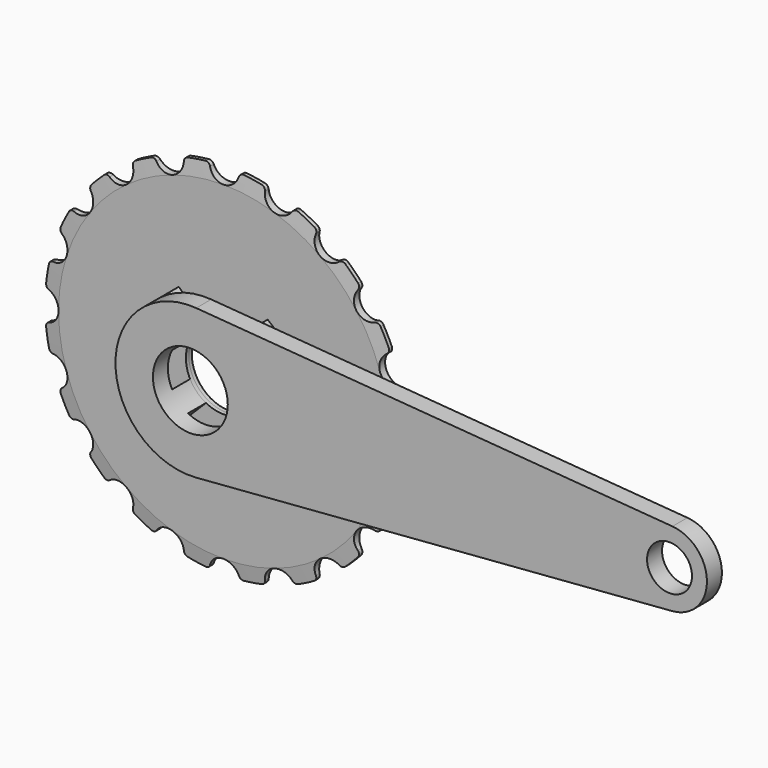
from build123d import *
from build123d import SkipClean  # not in build123d's __all__

# Parameters (mm, degrees)
F2_R          = 6.35
F3_DEPTH      = 1.5885
F3_DEPTH_BACK = 1.5885
F4_T1_DEPTH   = 10.5199898753
F5_R          = 15.875
F6_DEPTH      = 1.5885001
F6_DEPTH_BACK = 1.5885001
F8_D          = 5
F10_R         = 15.875
F10_R_2       = 9.525
F11_DEPTH     = 17.4625
F12_R         = 9.525
F12_R_2       = 15.875
F13_DEPTH     = 9.525
F15_DEPTH     = 9.525


# Not quite as in the source:
# - a fillet or chamfer that OpenCascade refuses, or shapes differently, is made with other operations: its cross-section is extruded or revolved along the edge and cut away or added


with BuildPart() as f1:
    # F0 (on Right) → F1 (revolve)
    with BuildSketch(Plane.YZ):
        Polygon((-0.79375, 76.2), (-1.5875, 69.85), (-1.5875, 0), (1.5875, 0), (1.5875, 69.85), (0.79375, 76.2), (0, 76.2), align=None)
    revolve(axis=Axis((0, -19.5679962635, 0), (0, -1, 0)))

    # F2 (on Front) → F3 (cut, two sides)
    with BuildSketch(Plane.XZ) as f3_sk:
        with Locations((0, 76.2)):
            Circle(F2_R)
        with Locations((-23.5470949714, 72.4705065417)):
            Circle(F2_R)
        with Locations((-44.7892362247, 61.6470949714)):
            Circle(F2_R)
        with Locations((-61.6470949714, 44.7892362247)):
            Circle(F2_R)
        with Locations((-72.4705065417, 23.5470949714)):
            Circle(F2_R)
        with Locations((-76.2, 0)):
            Circle(F2_R)
        with Locations((-72.4705065417, -23.5470949714)):
            Circle(F2_R)
        with Locations((-61.6470949714, -44.7892362247)):
            Circle(F2_R)
        with Locations((-44.7892362247, -61.6470949714)):
            Circle(F2_R)
        with Locations((-23.5470949714, -72.4705065417)):
            Circle(F2_R)
        with Locations((0, -76.2)):
            Circle(F2_R)
        with Locations((23.5470949714, -72.4705065417)):
            Circle(F2_R)
        with Locations((44.7892362247, -61.6470949714)):
            Circle(F2_R)
        with Locations((61.6470949714, -44.7892362247)):
            Circle(F2_R)
        with Locations((72.4705065417, -23.5470949714)):
            Circle(F2_R)
        with Locations((76.2, 0)):
            Circle(F2_R)
        with Locations((72.4705065417, 23.5470949714)):
            Circle(F2_R)
        with Locations((61.6470949714, 44.7892362247)):
            Circle(F2_R)
        with Locations((44.7892362247, 61.6470949714)):
            Circle(F2_R)
        with Locations((23.5470949714, 72.4705065417)):
            Circle(F2_R)
    extrude(amount=-F3_DEPTH, mode=Mode.SUBTRACT)
    extrude(f3_sk.sketch, amount=F3_DEPTH_BACK, mode=Mode.SUBTRACT)

    # F4: fillet of radius 1.905 on 40 edges, made by hand

    # F4_s2 → F4_t1 (cut)
    with BuildSketch(Plane.XZ.offset(-5.2599949376)):
        with BuildLine():
            ThreePointArc((-31.1382740919, 69.5474506116), (-29.8427555478, 69.6422506994), (-28.7876505623, 68.8845510068))
            ThreePointArc((-28.7876505623, 68.8845510068), (-29.185470054, 69.5496802154), (-29.4992984573, 70.258319013))
            ThreePointArc((-29.4992984573, 70.258319013), (-30.320869622, 69.9076881706), (-31.1382740919, 69.5474506116))
        make_face()
        with BuildLine():
            ThreePointArc((-17.1996246595, 72.6497288631), (-16.7913915004, 73.8828959411), (-15.6875728882, 74.5676877533))
            ThreePointArc((-15.6875728882, 74.5676877533), (-16.5606093201, 74.378667768), (-17.4313699926, 74.1794266639))
            ThreePointArc((-17.4313699926, 74.1794266639), (-17.2687350698, 73.4216621266), (-17.1996246595, 72.6497288631))
        make_face()
        with BuildLine():
            ThreePointArc((8.1229143268, 75.7658119658), (6.8615081353, 75.4556349604), (6.0921857451, 74.408974359))
            ThreePointArc((6.0921857451, 74.408974359), (6.264998336, 75.1644828106), (6.3444854527, 75.9354166667))
            ThreePointArc((6.3444854527, 75.9354166667), (7.2341969516, 75.8558263713), (8.1229143268, 75.7658119658))
        make_face()
        with BuildLine():
            ThreePointArc((-8.1229143268, 75.7658119658), (-6.8615081353, 75.4556349604), (-6.0921857451, 74.408974359))
            ThreePointArc((-6.0921857451, 74.408974359), (-6.264998336, 75.1644828106), (-6.3444854527, 75.9354166667))
            ThreePointArc((-6.3444854527, 75.9354166667), (-7.2341969516, 75.8558263713), (-8.1229143268, 75.7658119658))
        make_face()
        with BuildLine():
            ThreePointArc((-51.1056026357, 56.521300226), (-49.9027861206, 57.0117977139), (-48.6651795671, 56.6172278552))
            ThreePointArc((-48.6651795671, 56.6172278552), (-49.2490646159, 57.1268703396), (-49.7665145952, 57.7038475758))
            ThreePointArc((-49.7665145952, 57.7038475758), (-50.439524316, 57.1164983764), (-51.1056026357, 56.521300226))
        make_face()
        with BuildLine():
            ThreePointArc((-38.8078159657, 63.7790217256), (-38.8006327436, 65.0779842948), (-37.9624511672, 66.0703587199))
            ThreePointArc((-37.9624511672, 66.0703587199), (-38.734347767, 65.620806937), (-39.5009214915, 65.1622375408))
            ThreePointArc((-39.5009214915, 65.1622375408), (-39.1120843687, 64.4918175948), (-38.8078159657, 63.7790217256))
        make_face()
        with BuildLine():
            ThreePointArc((28.7876505623, 68.8845510068), (29.8427555478, 69.6422506994), (31.1382740919, 69.5474506116))
            ThreePointArc((31.1382740919, 69.5474506116), (30.320869622, 69.9076881706), (29.4992984573, 70.258319013))
            ThreePointArc((29.4992984573, 70.258319013), (29.185470054, 69.5496802154), (28.7876505623, 68.8845510068))
        make_face()
        with BuildLine():
            ThreePointArc((17.1996246595, 72.6497288631), (16.7913915004, 73.8828959411), (15.6875728882, 74.5676877533))
            ThreePointArc((15.6875728882, 74.5676877533), (16.5606093201, 74.378667768), (17.4313699926, 74.1794266639))
            ThreePointArc((17.4313699926, 74.1794266639), (17.2687350698, 73.4216621266), (17.1996246595, 72.6497288631))
        make_face()
        with BuildLine():
            ThreePointArc((48.6651795671, 56.6172278552), (49.9027861206, 57.0117977139), (51.1056026357, 56.521300226))
            ThreePointArc((51.1056026357, 56.521300226), (50.439524316, 57.1164983764), (49.7665145952, 57.7038475758))
            ThreePointArc((49.7665145952, 57.7038475758), (49.2490646159, 57.1268703396), (48.6651795671, 56.6172278552))
        make_face()
        with BuildLine():
            ThreePointArc((38.8078159657, 63.7790217256), (38.8006327436, 65.0779842948), (37.9624511672, 66.0703587199))
            ThreePointArc((37.9624511672, 66.0703587199), (38.734347767, 65.620806937), (39.5009214915, 65.1622375408))
            ThreePointArc((39.5009214915, 65.1622375408), (39.1120843687, 64.4918175948), (38.8078159657, 63.7790217256))
        make_face()
        with BuildLine():
            ThreePointArc((56.521300226, 51.1056026357), (57.0117977139, 49.9027861206), (56.6172278552, 48.6651795671))
            ThreePointArc((56.6172278552, 48.6651795671), (57.1268703396, 49.2490646159), (57.7038475758, 49.7665145952))
            ThreePointArc((57.7038475758, 49.7665145952), (57.1164983764, 50.439524316), (56.521300226, 51.1056026357))
        make_face()
        with BuildLine():
            ThreePointArc((63.7790217256, 38.8078159657), (65.0779842948, 38.8006327436), (66.0703587199, 37.9624511672))
            ThreePointArc((66.0703587199, 37.9624511672), (65.620806937, 38.734347767), (65.1622375408, 39.5009214915))
            ThreePointArc((65.1622375408, 39.5009214915), (64.4918175948, 39.1120843687), (63.7790217256, 38.8078159657))
        make_face()
        with BuildLine():
            ThreePointArc((-66.0703587199, 37.9624511672), (-65.0779842948, 38.8006327436), (-63.7790217256, 38.8078159657))
            ThreePointArc((-63.7790217256, 38.8078159657), (-64.4918175948, 39.1120843687), (-65.1622375408, 39.5009214915))
            ThreePointArc((-65.1622375408, 39.5009214915), (-65.620806937, 38.734347767), (-66.0703587199, 37.9624511672))
        make_face()
        with BuildLine():
            ThreePointArc((-56.6172278552, 48.6651795671), (-57.0117977139, 49.9027861206), (-56.521300226, 51.1056026357))
            ThreePointArc((-56.521300226, 51.1056026357), (-57.1164983764, 50.439524316), (-57.7038475758, 49.7665145952))
            ThreePointArc((-57.7038475758, 49.7665145952), (-57.1268703396, 49.2490646159), (-56.6172278552, 48.6651795671))
        make_face()
        with BuildLine():
            ThreePointArc((-74.5676877533, 15.6875728882), (-73.8828959411, 16.7913915004), (-72.6497288631, 17.1996246595))
            ThreePointArc((-72.6497288631, 17.1996246595), (-73.4216621266, 17.2687350698), (-74.1794266639, 17.4313699926))
            ThreePointArc((-74.1794266639, 17.4313699926), (-74.378667768, 16.5606093201), (-74.5676877533, 15.6875728882))
        make_face()
        with BuildLine():
            ThreePointArc((-68.8845510068, 28.7876505623), (-69.6422506994, 29.8427555478), (-69.5474506116, 31.1382740919))
            ThreePointArc((-69.5474506116, 31.1382740919), (-69.9076881706, 30.320869622), (-70.258319013, 29.4992984573))
            ThreePointArc((-70.258319013, 29.4992984573), (-69.5496802154, 29.185470054), (-68.8845510068, 28.7876505623))
        make_face()
        with BuildLine():
            ThreePointArc((-75.7658119658, -8.1229143268), (-75.4556349604, -6.8615081353), (-74.408974359, -6.0921857451))
            ThreePointArc((-74.408974359, -6.0921857451), (-75.1644828106, -6.264998336), (-75.9354166667, -6.3444854527))
            ThreePointArc((-75.9354166667, -6.3444854527), (-75.8558263713, -7.2341969516), (-75.7658119658, -8.1229143268))
        make_face()
        with BuildLine():
            ThreePointArc((-74.408974359, 6.0921857451), (-75.4556349604, 6.8615081353), (-75.7658119658, 8.1229143268))
            ThreePointArc((-75.7658119658, 8.1229143268), (-75.8558263713, 7.2341969516), (-75.9354166667, 6.3444854527))
            ThreePointArc((-75.9354166667, 6.3444854527), (-75.1644828106, 6.264998336), (-74.408974359, 6.0921857451))
        make_face()
        with BuildLine():
            ThreePointArc((-69.5474506116, -31.1382740919), (-69.6422506994, -29.8427555478), (-68.8845510068, -28.7876505623))
            ThreePointArc((-68.8845510068, -28.7876505623), (-69.5496802154, -29.185470054), (-70.258319013, -29.4992984573))
            ThreePointArc((-70.258319013, -29.4992984573), (-69.9076881706, -30.320869622), (-69.5474506116, -31.1382740919))
        make_face()
        with BuildLine():
            ThreePointArc((-72.6497288631, -17.1996246595), (-73.8828959411, -16.7913915004), (-74.5676877533, -15.6875728882))
            ThreePointArc((-74.5676877533, -15.6875728882), (-74.378667768, -16.5606093201), (-74.1794266639, -17.4313699926))
            ThreePointArc((-74.1794266639, -17.4313699926), (-73.4216621266, -17.2687350698), (-72.6497288631, -17.1996246595))
        make_face()
        with BuildLine():
            ThreePointArc((-56.521300226, -51.1056026357), (-57.0117977139, -49.9027861206), (-56.6172278552, -48.6651795671))
            ThreePointArc((-56.6172278552, -48.6651795671), (-57.1268703396, -49.2490646159), (-57.7038475758, -49.7665145952))
            ThreePointArc((-57.7038475758, -49.7665145952), (-57.1164983764, -50.439524316), (-56.521300226, -51.1056026357))
        make_face()
        with BuildLine():
            ThreePointArc((-63.7790217256, -38.8078159657), (-65.0779842948, -38.8006327436), (-66.0703587199, -37.9624511672))
            ThreePointArc((-66.0703587199, -37.9624511672), (-65.620806937, -38.734347767), (-65.1622375408, -39.5009214915))
            ThreePointArc((-65.1622375408, -39.5009214915), (-64.4918175948, -39.1120843687), (-63.7790217256, -38.8078159657))
        make_face()
        with BuildLine():
            ThreePointArc((-37.9624511672, -66.0703587199), (-38.8006327436, -65.0779842948), (-38.8078159657, -63.7790217256))
            ThreePointArc((-38.8078159657, -63.7790217256), (-39.1120843687, -64.4918175948), (-39.5009214915, -65.1622375408))
            ThreePointArc((-39.5009214915, -65.1622375408), (-38.734347767, -65.620806937), (-37.9624511672, -66.0703587199))
        make_face()
        with BuildLine():
            ThreePointArc((-48.6651795671, -56.6172278552), (-49.9027861206, -57.0117977139), (-51.1056026357, -56.521300226))
            ThreePointArc((-51.1056026357, -56.521300226), (-50.439524316, -57.1164983764), (-49.7665145952, -57.7038475758))
            ThreePointArc((-49.7665145952, -57.7038475758), (-49.2490646159, -57.1268703396), (-48.6651795671, -56.6172278552))
        make_face()
        with BuildLine():
            ThreePointArc((-15.6875728882, -74.5676877533), (-16.7913915004, -73.8828959411), (-17.1996246595, -72.6497288631))
            ThreePointArc((-17.1996246595, -72.6497288631), (-17.2687350698, -73.4216621266), (-17.4313699926, -74.1794266639))
            ThreePointArc((-17.4313699926, -74.1794266639), (-16.5606093201, -74.378667768), (-15.6875728882, -74.5676877533))
        make_face()
        with BuildLine():
            ThreePointArc((-28.7876505623, -68.8845510068), (-29.8427555478, -69.6422506994), (-31.1382740919, -69.5474506116))
            ThreePointArc((-31.1382740919, -69.5474506116), (-30.320869622, -69.9076881706), (-29.4992984573, -70.258319013))
            ThreePointArc((-29.4992984573, -70.258319013), (-29.185470054, -69.5496802154), (-28.7876505623, -68.8845510068))
        make_face()
        with BuildLine():
            ThreePointArc((8.1229143268, -75.7658119658), (6.8615081353, -75.4556349604), (6.0921857451, -74.408974359))
            ThreePointArc((6.0921857451, -74.408974359), (6.264998336, -75.1644828106), (6.3444854527, -75.9354166667))
            ThreePointArc((6.3444854527, -75.9354166667), (7.2341969516, -75.8558263713), (8.1229143268, -75.7658119658))
        make_face()
        with BuildLine():
            ThreePointArc((-6.0921857451, -74.408974359), (-6.8615081353, -75.4556349604), (-8.1229143268, -75.7658119658))
            ThreePointArc((-8.1229143268, -75.7658119658), (-7.2341969516, -75.8558263713), (-6.3444854527, -75.9354166667))
            ThreePointArc((-6.3444854527, -75.9354166667), (-6.264998336, -75.1644828106), (-6.0921857451, -74.408974359))
        make_face()
        with BuildLine():
            ThreePointArc((31.1382740919, -69.5474506116), (29.8427555478, -69.6422506994), (28.7876505623, -68.8845510068))
            ThreePointArc((28.7876505623, -68.8845510068), (29.185470054, -69.5496802154), (29.4992984573, -70.258319013))
            ThreePointArc((29.4992984573, -70.258319013), (30.320869622, -69.9076881706), (31.1382740919, -69.5474506116))
        make_face()
        with BuildLine():
            ThreePointArc((17.1996246595, -72.6497288631), (16.7913915004, -73.8828959411), (15.6875728882, -74.5676877533))
            ThreePointArc((15.6875728882, -74.5676877533), (16.5606093201, -74.378667768), (17.4313699926, -74.1794266639))
            ThreePointArc((17.4313699926, -74.1794266639), (17.2687350698, -73.4216621266), (17.1996246595, -72.6497288631))
        make_face()
        with BuildLine():
            ThreePointArc((51.1056026357, -56.521300226), (49.9027861206, -57.0117977139), (48.6651795671, -56.6172278552))
            ThreePointArc((48.6651795671, -56.6172278552), (49.2490646159, -57.1268703396), (49.7665145952, -57.7038475758))
            ThreePointArc((49.7665145952, -57.7038475758), (50.439524316, -57.1164983764), (51.1056026357, -56.521300226))
        make_face()
        with BuildLine():
            ThreePointArc((38.8078159657, -63.7790217256), (38.8006327436, -65.0779842948), (37.9624511672, -66.0703587199))
            ThreePointArc((37.9624511672, -66.0703587199), (38.734347767, -65.620806937), (39.5009214915, -65.1622375408))
            ThreePointArc((39.5009214915, -65.1622375408), (39.1120843687, -64.4918175948), (38.8078159657, -63.7790217256))
        make_face()
        with BuildLine():
            ThreePointArc((66.0703587199, -37.9624511672), (65.0779842948, -38.8006327436), (63.7790217256, -38.8078159657))
            ThreePointArc((63.7790217256, -38.8078159657), (64.4918175948, -39.1120843687), (65.1622375408, -39.5009214915))
            ThreePointArc((65.1622375408, -39.5009214915), (65.620806937, -38.734347767), (66.0703587199, -37.9624511672))
        make_face()
        with BuildLine():
            ThreePointArc((56.6172278552, -48.6651795671), (57.0117977139, -49.9027861206), (56.521300226, -51.1056026357))
            ThreePointArc((56.521300226, -51.1056026357), (57.1164983764, -50.439524316), (57.7038475758, -49.7665145952))
            ThreePointArc((57.7038475758, -49.7665145952), (57.1268703396, -49.2490646159), (56.6172278552, -48.6651795671))
        make_face()
        with BuildLine():
            ThreePointArc((74.5676877533, -15.6875728882), (73.8828959411, -16.7913915004), (72.6497288631, -17.1996246595))
            ThreePointArc((72.6497288631, -17.1996246595), (73.4216621266, -17.2687350698), (74.1794266639, -17.4313699926))
            ThreePointArc((74.1794266639, -17.4313699926), (74.378667768, -16.5606093201), (74.5676877533, -15.6875728882))
        make_face()
        with BuildLine():
            ThreePointArc((68.8845510068, -28.7876505623), (69.6422506994, -29.8427555478), (69.5474506116, -31.1382740919))
            ThreePointArc((69.5474506116, -31.1382740919), (69.9076881706, -30.320869622), (70.258319013, -29.4992984573))
            ThreePointArc((70.258319013, -29.4992984573), (69.5496802154, -29.185470054), (68.8845510068, -28.7876505623))
        make_face()
        with BuildLine():
            ThreePointArc((69.5474506116, 31.1382740919), (69.6422506994, 29.8427555478), (68.8845510068, 28.7876505623))
            ThreePointArc((68.8845510068, 28.7876505623), (69.5496802154, 29.185470054), (70.258319013, 29.4992984573))
            ThreePointArc((70.258319013, 29.4992984573), (69.9076881706, 30.320869622), (69.5474506116, 31.1382740919))
        make_face()
        with BuildLine():
            ThreePointArc((72.6497288631, 17.1996246595), (73.8828959411, 16.7913915004), (74.5676877533, 15.6875728882))
            ThreePointArc((74.5676877533, 15.6875728882), (74.378667768, 16.5606093201), (74.1794266639, 17.4313699926))
            ThreePointArc((74.1794266639, 17.4313699926), (73.4216621266, 17.2687350698), (72.6497288631, 17.1996246595))
        make_face()
        with BuildLine():
            ThreePointArc((75.7658119658, 8.1229143268), (75.4556349604, 6.8615081353), (74.408974359, 6.0921857451))
            ThreePointArc((74.408974359, 6.0921857451), (75.1644828106, 6.264998336), (75.9354166667, 6.3444854527))
            ThreePointArc((75.9354166667, 6.3444854527), (75.8558263713, 7.2341969516), (75.7658119658, 8.1229143268))
        make_face()
        with BuildLine():
            ThreePointArc((74.408974359, -6.0921857451), (75.4556349604, -6.8615081353), (75.7658119658, -8.1229143268))
            ThreePointArc((75.7658119658, -8.1229143268), (75.8558263713, -7.2341969516), (75.9354166667, -6.3444854527))
            ThreePointArc((75.9354166667, -6.3444854527), (75.1644828106, -6.264998336), (74.408974359, -6.0921857451))
        make_face()
    extrude(amount=F4_T1_DEPTH, mode=Mode.SUBTRACT)

    # F5 (on Front) → F6 (cut, two sides)
    with BuildSketch(Plane.XZ) as f6_sk:
        Circle(F5_R)
    extrude(amount=-F6_DEPTH, mode=Mode.SUBTRACT)
    extrude(f6_sk.sketch, amount=F6_DEPTH_BACK, mode=Mode.SUBTRACT)

    # F8 (through all)
    with Locations(Plane.XZ.offset(1.5875)):
        with Locations((-17.9605122421, 17.9605122421), (17.9605122421, 17.9605122421), (17.9605122421, -17.9605122421), (-17.9605122421, -17.9605122421)):
            Hole(F8_D / 2)


with BuildPart() as f11:
    # F10 (on offset) → F11 (new body, through all)
    with BuildSketch(Plane.XZ.offset(19.05)):
        with BuildLine():
            ThreePointArc((2.48046875, -31.6529583891), (23.3111280595, -21.5558300372), (31.75, 0))
            ThreePointArc((31.75, 0), (23.3111280595, 21.5558300372), (2.48046875, 31.6529583891))
            ThreePointArc((2.48046875, 31.6529583891), (-31.75, 0), (2.48046875, -31.6529583891))
        make_face()
        Circle(F10_R, mode=Mode.SUBTRACT)
        with BuildLine():
            ThreePointArc((2.48046875, 31.6529583891), (23.3111280595, 21.5558300372), (31.75, 0))
            ThreePointArc((31.75, 0), (23.3111280595, -21.5558300372), (2.48046875, -31.6529583891))
            Line((2.48046875, -31.6529583891), (204.440234375, -15.8264791945))
            ThreePointArc((204.440234375, -15.8264791945), (187.325, 0), (204.440234375, 15.8264791945))
            Line((204.440234375, 15.8264791945), (2.48046875, 31.6529583891))
        make_face()
        with BuildLine():
            ThreePointArc((219.075, 0), (214.8555640297, 10.7779150186), (204.440234375, 15.8264791945))
            ThreePointArc((204.440234375, 15.8264791945), (187.325, 0), (204.440234375, -15.8264791945))
            ThreePointArc((204.440234375, -15.8264791945), (214.8555640297, -10.7779150186), (219.075, 0))
        make_face()
        with Locations((203.2, 0)):
            Circle(F10_R_2, mode=Mode.SUBTRACT)
    extrude(amount=-F11_DEPTH)

    # F12 (on face) → F13 (cut)
    with BuildSketch(Plane(origin=(0, -1.5875, 0), x_dir=(-1, 0, 0), z_dir=(0, 1, 0))):
        with BuildLine():
            Line((-2.48046875, 31.6529583891), (-204.440234375, 15.8264791945))
            ThreePointArc((-204.440234375, 15.8264791945), (-187.325, 0), (-204.440234375, -15.8264791945))
            Line((-204.440234375, -15.8264791945), (-2.48046875, -31.6529583891))
            ThreePointArc((-2.48046875, -31.6529583891), (-31.75, 0), (-2.48046875, 31.6529583891))
        make_face()
        with BuildLine():
            ThreePointArc((-204.440234375, -15.8264791945), (-187.325, 0), (-204.440234375, 15.8264791945))
            ThreePointArc((-204.440234375, 15.8264791945), (-219.075, 0), (-204.440234375, -15.8264791945))
        make_face()
        with Locations((-203.2, 0)):
            Circle(F12_R, mode=Mode.SUBTRACT)
        Circle(F12_R_2)
        with Locations((-203.2, 0)):
            Circle(F12_R)
    with SkipClean():  # cleaning this boolean's faces spoils the solid; the shape is the same uncleaned
        extrude(amount=-F13_DEPTH, mode=Mode.SUBTRACT)

    # F14 (on face) → F15 (cut, through all)
    with BuildSketch(Plane(origin=(0, -1.5875, 0), x_dir=(-1, 0, 0), z_dir=(0, 1, 0))):
        with BuildLine():
            ThreePointArc((-7.3406768954, 14.0758689862), (0, 15.875), (7.3406768954, 14.0758689862))
            Line((7.3406768954, 14.0758689862), (18.829037638, 25.5642297288))
            ThreePointArc((18.829037638, 25.5642297288), (8.7227908576, 30.5282724643), (-2.48046875, 31.6529583891))
            ThreePointArc((-2.48046875, 31.6529583891), (-11.0811515557, 29.7534969407), (-18.829037638, 25.5642297288))
            Line((-18.829037638, 25.5642297288), (-7.3406768954, 14.0758689862))
        make_face()
        with BuildLine():
            ThreePointArc((-15.875, 0), (-15.4186582613, 3.7789684336), (-14.0758689862, 7.3406768954))
            Line((-14.0758689862, 7.3406768954), (-25.5642297288, 18.829037638))
            ThreePointArc((-25.5642297288, 18.829037638), (-31.75, 0), (-25.5642297288, -18.829037638))
            Line((-25.5642297288, -18.829037638), (-14.0758689862, -7.3406768954))
            ThreePointArc((-14.0758689862, -7.3406768954), (-15.4186582613, -3.7789684336), (-15.875, 0))
        make_face()
        with BuildLine():
            Line((18.829037638, -25.5642297288), (7.3406768954, -14.0758689862))
            ThreePointArc((7.3406768954, -14.0758689862), (0, -15.875), (-7.3406768954, -14.0758689862))
            Line((-7.3406768954, -14.0758689862), (-18.829037638, -25.5642297288))
            ThreePointArc((-18.829037638, -25.5642297288), (-11.0811515557, -29.7534969407), (-2.48046875, -31.6529583891))
            ThreePointArc((-2.48046875, -31.6529583891), (8.7227908576, -30.5282724643), (18.829037638, -25.5642297288))
        make_face()
        with BuildLine():
            ThreePointArc((14.0758689862, 7.3406768954), (15.4186582613, 3.7789684336), (15.875, 0))
            ThreePointArc((15.875, 0), (15.4186582613, -3.7789684336), (14.0758689862, -7.3406768954))
            Line((14.0758689862, -7.3406768954), (25.5642297288, -18.829037638))
            ThreePointArc((25.5642297288, -18.829037638), (30.1639419994, -9.909546057), (31.75, 0))
            ThreePointArc((31.75, 0), (30.1639419994, 9.909546057), (25.5642297288, 18.829037638))
            Line((25.5642297288, 18.829037638), (14.0758689862, 7.3406768954))
        make_face()
    extrude(amount=-F15_DEPTH, mode=Mode.SUBTRACT)


solid = Compound([f1.part, f11.part])
